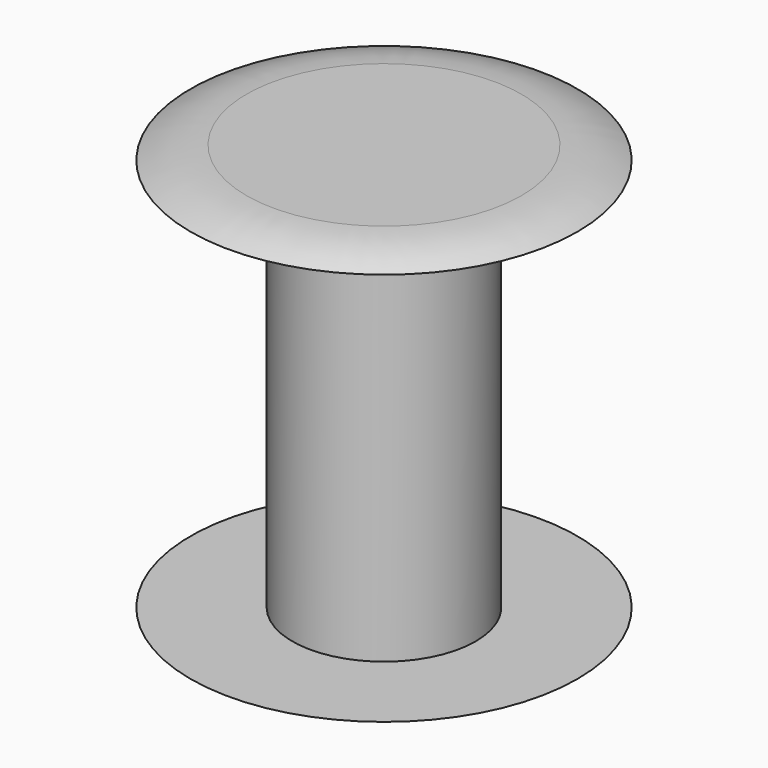
from build123d import *

# Parameters (mm, degrees)
F0_W = 1.905
F0_H = 0.254


# Not quite as in the source:
# - a fillet or chamfer that OpenCascade refuses, or shapes differently, is made with other operations: its cross-section is extruded or revolved along the edge and cut away or added


with BuildPart() as f1:
    # F0 (on Front) → F1 (revolve)
    with BuildSketch(Plane.XZ):
        with Locations((-29.5277546042, 20.4458203979)):
            Rectangle(F0_W, F0_H)
        Polygon((-30.4802546042, 20.3188203979), (-30.4802546042, 20.5728203979), (-32.1947546042, 20.5728203979), (-32.1947546042, 12.6988203979), (-30.4802546042, 12.6988203979), (-30.4802546042, 12.9528203979), align=None)
        with Locations((-29.5277546042, 12.8258203979)):
            Rectangle(F0_W, F0_H)
    revolve(axis=Axis((-32.1947546042, 0, 16.6358203979), (0, 0, 1)))

    # F2: fillet of radius 2.286 on 1 edges, made by hand

    # F2_s1 → F2_t2 (revolve, cut)
    with BuildSketch(Plane.XZ):
        with BuildLine():
            ThreePointArc((-29.6225234331, 20.5728203979), (-29.0837080659, 20.5084130698), (-28.5752546042, 20.3188203979))
            Line((-28.5752546042, 20.3188203979), (-28.5752546042, 20.5728203979))
            Line((-28.5752546042, 20.5728203979), (-29.6225234331, 20.5728203979))
        make_face()
    revolve(axis=Axis((-32.1947546042, 0, 20.5728203979), (0, 0, 1)), mode=Mode.SUBTRACT)

    # F3: fillet of radius 2.286 on 1 edges, made by hand

    # F3_s1 → F3_t2 (revolve, cut)
    with BuildSketch(Plane.XZ):
        with BuildLine():
            ThreePointArc((-28.5752546042, 12.9528203979), (-29.0837080659, 12.763227726), (-29.6225234331, 12.6988203979))
            Line((-29.6225234331, 12.6988203979), (-28.5752546042, 12.6988203979))
            Line((-28.5752546042, 12.6988203979), (-28.5752546042, 12.9528203979))
        make_face()
    revolve(axis=Axis((-32.1947546042, 0, 12.6988203979), (0, 0, 1)), mode=Mode.SUBTRACT)


solid = f1.part
